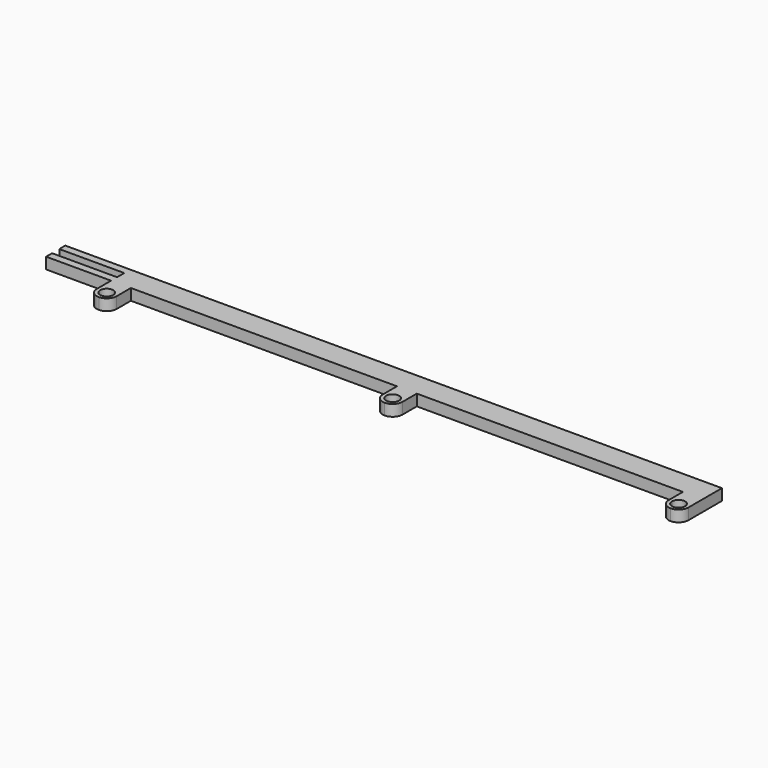
from build123d import *

# Parameters (mm, degrees)
F0_W     = 259.72
F0_H     = 6.4
F1_DEPTH = 3
F3_DEPTH = 3
F4_R     = 2.63999
F5_W     = 17.32
F5_H     = 2.4
F6_DEPTH = 3.001


# Not quite as in the source:
# - a fillet or chamfer is up to 0.001 mm smaller than in the source, because OpenCascade refuses the exact size


with BuildPart() as f1:
    # F0 (on Top) → F1 (new body)
    with BuildSketch(Plane.XY):
        Rectangle(F0_W, F0_H)
    extrude(amount=F1_DEPTH)

    # F2 (on Top) → F3 (join)
    with BuildSketch(Plane.XY):
        with BuildLine():
            Line((129.86, -10.59), (129.86, -3.2))
            Line((129.86, -3.2), (124.58, -3.2))
            Line((124.58, -3.2), (124.58, -7.95))
            Line((124.58, -7.95), (125.47, -7.95))
            ThreePointArc((125.47, -7.95), (127.22, -6.2), (128.97, -7.95))
            ThreePointArc((128.97, -7.95), (128.4574368671, -9.1874368671), (127.22, -9.7))
            Line((127.22, -9.7), (127.22, -10.59))
            Line((127.22, -10.59), (129.86, -10.59))
        make_face()
        with BuildLine():
            Line((125.47, -7.95), (124.58, -7.95))
            Line((124.58, -7.95), (124.58, -10.59))
            Line((124.58, -10.59), (127.22, -10.59))
            Line((127.22, -10.59), (127.22, -9.7))
            ThreePointArc((127.22, -9.7), (125.9825631329, -9.1874368671), (125.47, -7.95))
        make_face()
        Polygon((53.66, -10.59), (53.66, -3.2), (48.38, -3.2), (48.38, -7.95), (48.38, -10.59), align=None)
        with BuildLine():
            ThreePointArc((52.77, -7.95), (51.02, -9.7), (49.27, -7.95))
            ThreePointArc((49.27, -7.95), (51.02, -6.2), (52.77, -7.95))
        make_face(mode=Mode.SUBTRACT)
        Polygon((-22.54, -3.2), (-27.82, -3.2), (-27.82, -7.95), (-27.82, -10.59), (-22.54, -10.59), align=None)
        with BuildLine():
            ThreePointArc((-23.43, -7.95), (-25.18, -9.7), (-26.93, -7.95))
            ThreePointArc((-26.93, -7.95), (-25.18, -6.2), (-23.43, -7.95))
        make_face(mode=Mode.SUBTRACT)
    extrude(amount=F3_DEPTH)

    # F4 (radius 2.64 in the source; OpenCascade refuses exactly that, so slightly less here)
    f4_edges = [f1.edges().sort_by_distance(p)[0] for p in [
        (48.38, -10.59, 1.5),
        (53.66, -10.59, 1.5),
        (124.58, -10.59, 1.5),
        (129.86, -10.59, 1.5),
        (-27.82, -10.59, 1.5),
        (-22.54, -10.59, 1.5),
    ]]
    fillet(f4_edges, radius=F4_R)

    # F5 (on face) → F6 (cut, through all)
    with BuildSketch(Plane.XY.offset(3)):
        Polygon((-45.14, 3.2), (-129.86, 3.2), (-129.86, -3.2), (-45.14, -3.2), (-45.14, -1.2), (-45.14, 1.2), align=None)
        with Locations((-36.48, 0)):
            Rectangle(F5_W, F5_H)
    extrude(amount=-F6_DEPTH, mode=Mode.SUBTRACT)


solid = f1.part
